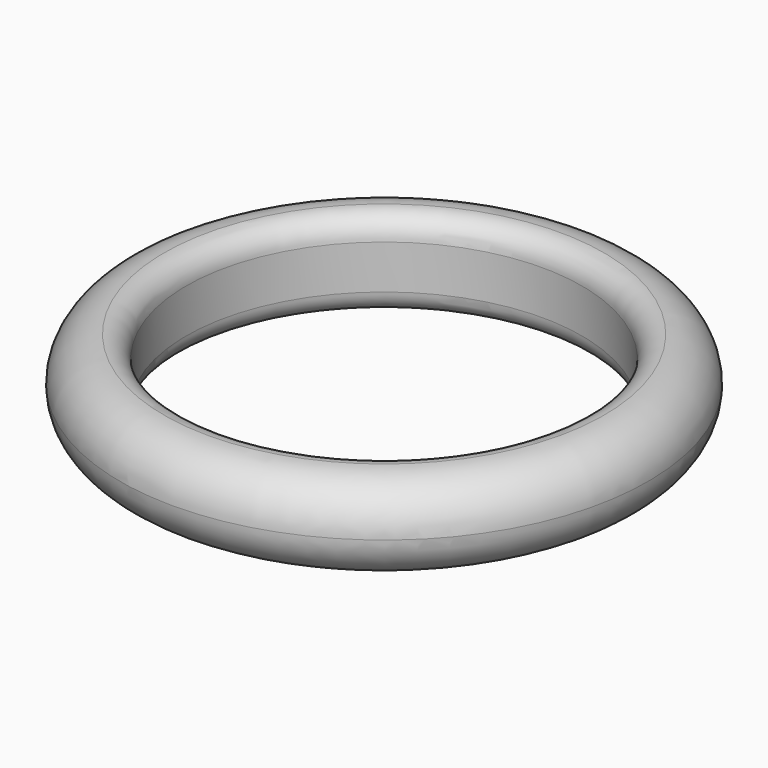
from build123d import *

# Parameters (mm, degrees)
F0_W = 3
F0_H = 4
F2_R = 1.99999
F3_R = 1


# Not quite as in the source:
# - a fillet or chamfer is up to 0.001 mm smaller than in the source, because OpenCascade refuses the exact size


with BuildPart() as f1:
    # F0 (on Right) → F1 (revolve)
    with BuildSketch(Plane.YZ):
        with Locations((-10.5, 2)):
            Rectangle(F0_W, F0_H)
    revolve(axis=Axis((0, 0, 2.5232175078), (0, 0, 1)))

    # F2 (radius 2 in the source; OpenCascade refuses exactly that, so slightly less here)
    f2_edges = [f1.edges().sort_by_distance(p)[0] for p in [
        (0, 12, 0),
        (0, 12, 4),
    ]]
    fillet(f2_edges, radius=F2_R)

    # F3
    f3_edges = [f1.edges().sort_by_distance(p)[0] for p in [
        (0, 9, 0),
        (0, 9, 4),
    ]]
    fillet(f3_edges, radius=F3_R)


solid = f1.part
